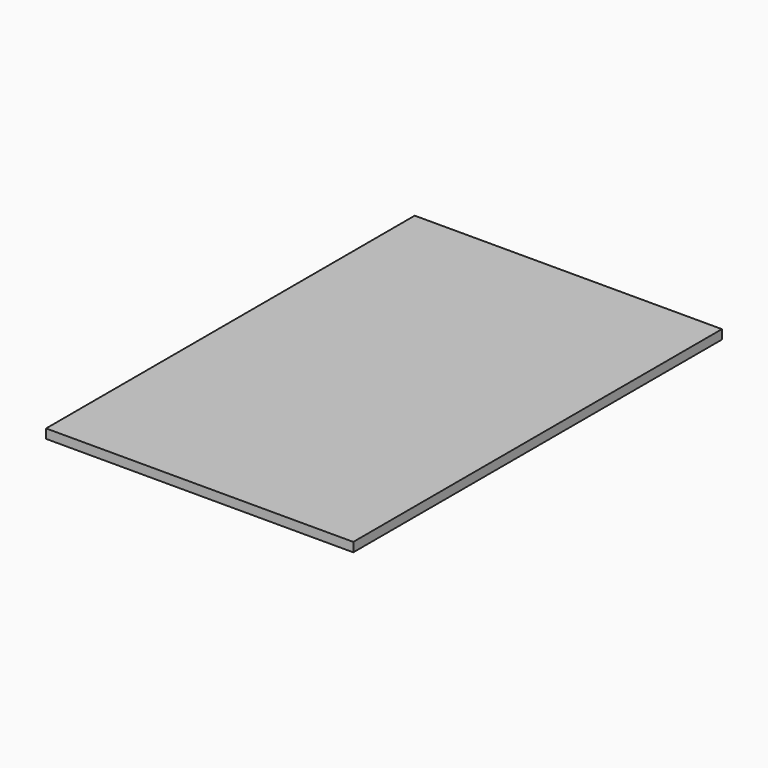
from build123d import *

# Parameters (mm, degrees)
F0_W     = 1000
F0_H     = 1500
F1_DEPTH = 30


# Not quite as in the source:
# - a feature of the source that left no trace in its solid (it failed there, or was rolled back) is left out


with BuildPart() as f1:
    # F0 (on Top) → F1 (new body)
    with BuildSketch(Plane.XY):
        Rectangle(F0_W, F0_H)
    extrude(amount=F1_DEPTH)


solid = f1.part
